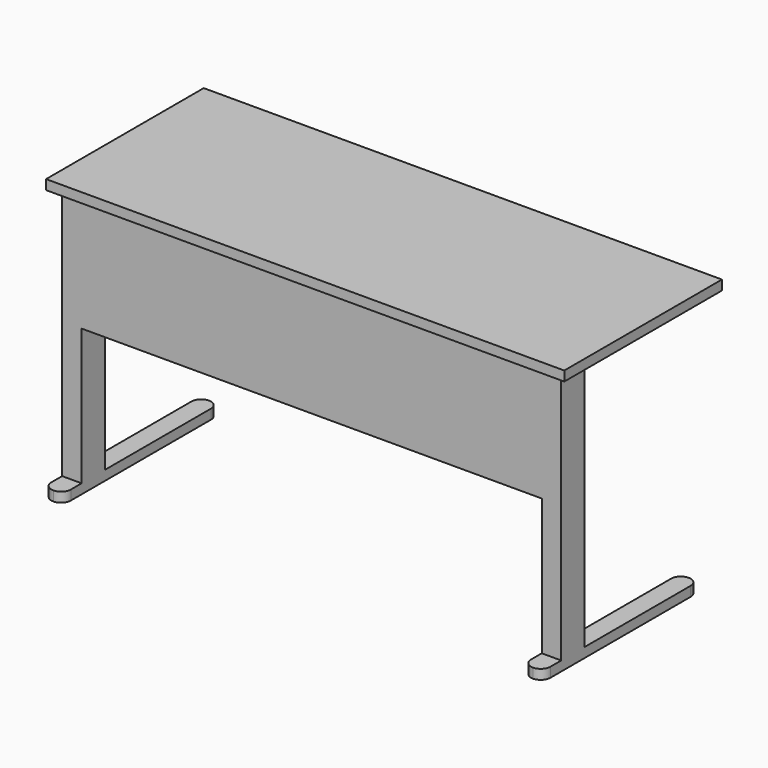
from build123d import *

# Parameters (mm, degrees)
F0_W      = 1352.55
F0_H      = 514.35
F1_DEPTH  = 25.4
F2_W      = 50.8
F2_H      = 317.5
F3_DEPTH  = 38.1
F4_W      = 50.8
F4_H      = 76.2
F5_DEPTH  = 660.4
F6_W      = 50.8
F6_H      = 508
F7_DEPTH  = 25.4
F8_R      = 25.4
F9_R      = 25.39999
F10_R     = 25.4
F11_R     = 25.39999
F12_R     = 25.39999
F13_R     = 25.39999
F14_W     = 1201.120785141
F14_H     = 25.4
F15_DEPTH = 304.8


# Not quite as in the source:
# - a fillet or chamfer is up to 0.001 mm smaller than in the source, because OpenCascade refuses the exact size


with BuildPart() as f1:
    # F0 (on Top) → F1 (new body)
    with BuildSketch(Plane.XY):
        with Locations((3.3097676933, -84.2684167102)):
            Rectangle(F0_W, F0_H)
    extrude(amount=F1_DEPTH)

    # F2 (on face) → F3 (join)
    with BuildSketch(Plane.XY.offset(25.4)):
        with Locations((-625.9603925705, -81.0934167102)):
            Rectangle(F2_W, F2_H)
        with Locations((625.9603925705, -81.0934167102)):
            Rectangle(F2_W, F2_H)
    extrude(amount=-F3_DEPTH)

    # F4 (on face) → F5 (join)
    with BuildSketch(Plane(origin=(0, 0, 0), x_dir=(1, 0, 0), z_dir=(0, 0, -1))):
        with Locations((-625.9603925705, 277.9434167102)):
            Rectangle(F4_W, F4_H)
        with Locations((625.9603925705, 277.9434167102)):
            Rectangle(F4_W, F4_H)
    extrude(amount=F5_DEPTH)

    # F6 (on face) → F7 (join)
    with BuildSketch(Plane(origin=(0, 0, -660.4), x_dir=(1, 0, 0), z_dir=(0, 0, -1))):
        with Locations((625.9603925705, 122.6374032485)):
            Rectangle(F6_W, F6_H)
        with Locations((-625.9603925705, 122.6374032485)):
            Rectangle(F6_W, F6_H)
    extrude(amount=F7_DEPTH)

    # F8
    f8_edges = [f1.edges().sort_by_distance(p)[0] for p in [
        (651.360393, 131.362597, -673.1),
    ]]
    fillet(f8_edges, radius=F8_R)

    # F9 (radius 25.4 in the source; OpenCascade refuses exactly that, so slightly less here)
    f9_edges = [f1.edges().sort_by_distance(p)[0] for p in [
        (600.560393, 131.362597, -673.1),
    ]]
    fillet(f9_edges, radius=F9_R)

    # F10
    f10_edges = [f1.edges().sort_by_distance(p)[0] for p in [
        (651.360393, -376.637403, -673.1),
    ]]
    fillet(f10_edges, radius=F10_R)

    # F11 (radius 25.4 in the source; OpenCascade refuses exactly that, so slightly less here)
    f11_edges = [f1.edges().sort_by_distance(p)[0] for p in [
        (600.560393, -376.637403, -673.1),
    ]]
    fillet(f11_edges, radius=F11_R)

    # F12 (radius 25.4 in the source; OpenCascade refuses exactly that, so slightly less here)
    f12_edges = [f1.edges().sort_by_distance(p)[0] for p in [
        (-600.560393, -376.637403, -673.1),
        (-651.360393, -376.637403, -673.1),
    ]]
    fillet(f12_edges, radius=F12_R)

    # F13 (radius 25.4 in the source; OpenCascade refuses exactly that, so slightly less here)
    f13_edges = [f1.edges().sort_by_distance(p)[0] for p in [
        (-651.360393, 131.362597, -673.1),
        (-600.560393, 131.362597, -673.1),
    ]]
    fillet(f13_edges, radius=F13_R)

    # F14 (on face) → F15 (join)
    with BuildSketch(Plane(origin=(0, 0, 0), x_dir=(1, 0, 0), z_dir=(0, 0, -1))):
        with Locations((0, 303.3434167102)):
            Rectangle(F14_W, F14_H)
    extrude(amount=F15_DEPTH)


solid = f1.part
